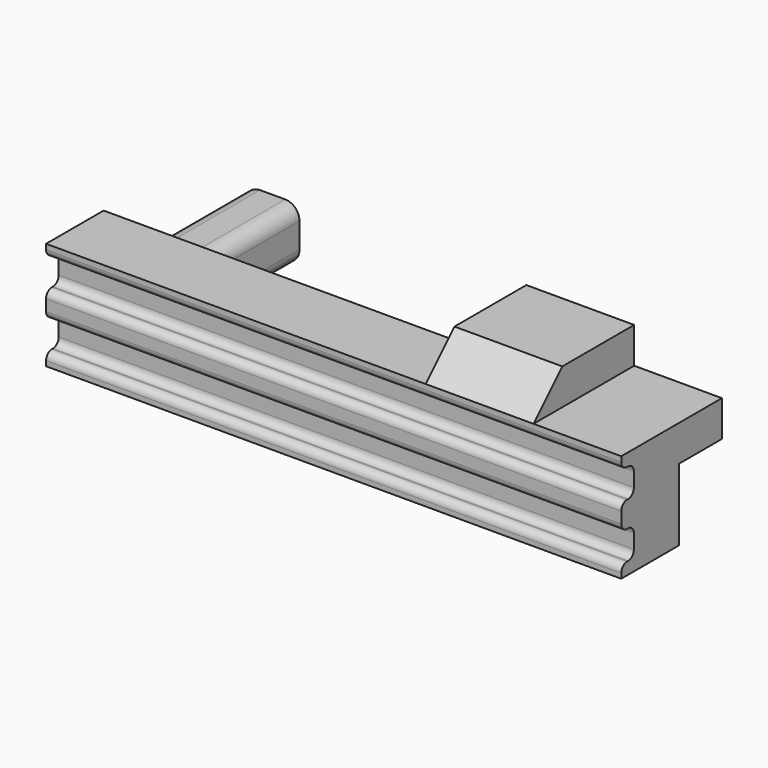
from build123d import *

# Parameters (mm, degrees)
F0_W      = 50.8
F0_H      = 9.525
F1_DEPTH  = 3.175
F2_W      = 3.175
F2_H      = 9.525
F3_DEPTH  = 50.8
F4_W      = 4.7625
F4_H      = 4.7625
F5_DEPTH  = 12.7
F6_R      = 1.27
F7_W      = 9.525
F7_H      = 3.175
F8_DEPTH  = 3.175
F9_W      = 17.272898303
F9_H      = 3.175
F9_W_2    = 9.525
F10_DEPTH = 4.7625
F11_W     = 1.3907738797
F11_H     = 2.54
F12_DEPTH = 50.8
F13_R     = 0.635
F14_SIZE  = 3.17499


# Not quite as in the source:
# - a fillet or chamfer is up to 0.001 mm smaller than in the source, because OpenCascade refuses the exact size


with BuildPart() as f1:
    # F0 (on Front) → F1 (new body)
    with BuildSketch(Plane.XZ):
        Rectangle(F0_W, F0_H)
    extrude(amount=F1_DEPTH)

    # F2 (on face) → F3 (join)
    with BuildSketch(Plane.YZ.offset(25.4)):
        with Locations((-4.7625, 0)):
            Rectangle(F2_W, F2_H)
    extrude(amount=-F3_DEPTH)

    # F4 (on face) → F5 (join)
    with BuildSketch(Plane(origin=(0, 0, 0), x_dir=(-1, 0, 0), z_dir=(0, 1, 0))):
        with Locations((20.6375, 0)):
            Rectangle(F4_W, F4_H)
    extrude(amount=F5_DEPTH)

    # F6
    f6_edges = [f1.edges().sort_by_distance(p)[0] for p in [
        (-18.25625, 6.35, 2.38125),
        (-23.01875, 6.35, 2.38125),
        (-18.25625, 6.35, -2.38125),
        (-23.01875, 6.35, -2.38125),
    ]]
    fillet(f6_edges, radius=F6_R)

    # F7 (on face) → F8 (join)
    with BuildSketch(Plane.XY.offset(4.7625)):
        with Locations((12.889601697, -1.5875)):
            Rectangle(F7_W, F7_H)
    extrude(amount=F8_DEPTH)

    # F9 (on face) → F10 (join)
    with BuildSketch(Plane(origin=(0, 0, 0), x_dir=(-1, 0, 0), z_dir=(0, 1, 0))):
        with Locations((-16.7635508485, 3.175)):
            Rectangle(F9_W, F9_H)
        with Locations((-12.889601697, 6.35)):
            Rectangle(F9_W_2, F9_H)
    extrude(amount=F10_DEPTH)

    # F11 (on face) → F12 (cut)
    with BuildSketch(Plane.YZ.offset(25.4)):
        with Locations((-5.6546130601, 2.3944999478)):
            Rectangle(F11_W, F11_H)
        with Locations((-5.6546130601, -2.4159172396)):
            Rectangle(F11_W, F11_H)
    extrude(amount=-F12_DEPTH, mode=Mode.SUBTRACT)

    # F13
    f13_edges = [f1.edges().sort_by_distance(p)[0] for p in [
        (0, -4.959226, 1.1245),
        (0, -4.959226, 3.6645),
        (0, -4.959226, -3.685917),
        (0, -4.959226, -1.145917),
        (0, -6.35, 1.1245),
        (0, -6.35, -1.145917),
        (0, -6.35, 3.6645),
        (0, -6.35, -3.685917),
    ]]
    fillet(f13_edges, radius=F13_R)

    # F14 (size 3.175 in the source; OpenCascade refuses exactly that, so slightly less here)
    f14_edges = [f1.edges().sort_by_distance(p)[0] for p in [
        (12.889602, -3.175, 4.7625),
    ]]
    chamfer(f14_edges, length=F14_SIZE)


solid = f1.part
